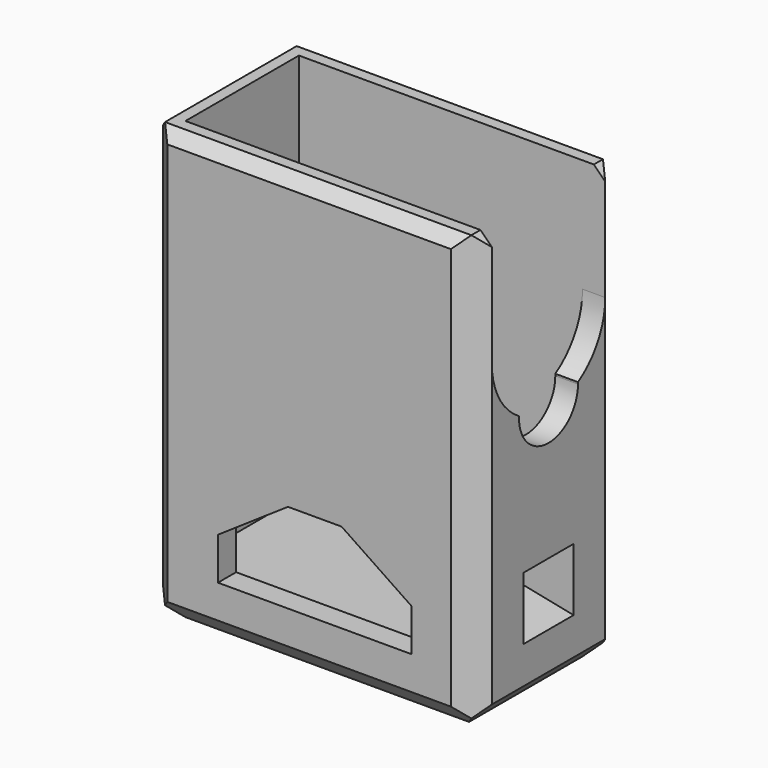
from build123d import *

# Parameters (mm, degrees)
F0_W      = 29
F0_H      = 16.5
F1_DEPTH  = 38.5
F2_T      = -2
F3_DEPTH  = 2.25
F4_SIZE   = 2
F5_SIZE   = 2
F6_SIZE   = 0.99999
F8_DEPTH  = 16.501
F10_DEPTH = 2
F11_R     = 2
F12_DEPTH = 2.001
F13_W     = 7.54
F13_H     = 7.25
F13_R     = 1.1
F14_DEPTH = 6.35
F17_W     = 5.481
F17_H     = 4.583
F15_W     = 5.538
F15_H     = 5.533


# Not quite as in the source:
# - a fillet or chamfer is up to 0.001 mm smaller than in the source, because OpenCascade refuses the exact size


with BuildPart() as f1:
    # F0 (on Top) → F1 (new body)
    with BuildSketch(Plane.XY):
        with Locations((14.5, 8.25)):
            Rectangle(F0_W, F0_H)
    extrude(amount=F1_DEPTH)

    # F2
    f2_openings = [f1.faces().sort_by_distance(p)[0] for p in [
        (14.5, 8.25, 38.5),
    ]]
    offset(amount=F2_T, openings=f2_openings)

    # F3 (add): a face of the model
    f3_faces = [f1.faces().sort_by_distance(p)[0] for p in [
        (14.5, 8.25, 2),
    ]]
    extrude(f3_faces, amount=F3_DEPTH)

    # F4
    f4_edges = [f1.edges().sort_by_distance(p)[0] for p in [
        (29, 0, 19.25),
        (29, 16.5, 19.25),
        (0, 16.5, 19.25),
        (0, 0, 19.25),
    ]]
    chamfer(f4_edges, length=F4_SIZE)

    # F5 (call 1 of 4: OpenCascade refuses the feature's edges together)
    f5_edges = [f1.edges().sort_by_distance(p)[0] for p in [
        (14.5, 16.5, 0),
    ]]
    chamfer(f5_edges, length=F5_SIZE)

    # F5#2 (call 2 of 4)
    f5_2_edges = [f1.edges().sort_by_distance(p)[0] for p in [
        (0, 8.25, 0),
    ]]
    chamfer(f5_2_edges, length=F5_SIZE)

    # F5#3 (call 3 of 4)
    f5_3_edges = [f1.edges().sort_by_distance(p)[0] for p in [
        (14.5, 0, 0),
    ]]
    chamfer(f5_3_edges, length=F5_SIZE)

    # F5#4 (call 4 of 4)
    f5_4_edges = [f1.edges().sort_by_distance(p)[0] for p in [
        (29, 8.25, 0),
    ]]
    chamfer(f5_4_edges, length=F5_SIZE)

    # F6 (size 1 in the source; OpenCascade refuses exactly that, so slightly less here)
    f6_edges = [f1.edges().sort_by_distance(p)[0] for p in [
        (14.5, 16.5, 38.5),
        (0, 8.25, 38.5),
        (14.5, 0, 38.5),
        (29, 8.25, 38.5),
    ]]
    chamfer(f6_edges, length=F6_SIZE)

    # F7 (on face) → F8 (cut, through all)
    with BuildSketch(Plane.XZ):
        Polygon((6.464, 8.664), (6.464, 4.94), (23.536, 4.94), (23.536, 8.664), (17.364, 12.834), (12.635, 12.834), align=None)
    extrude(amount=-F8_DEPTH, mode=Mode.SUBTRACT)

    # F9 (on face) → F10 (cut, through all)
    with BuildSketch(Plane.YZ.offset(29)):
        with BuildLine():
            Line((14.5, 38.5), (2, 38.5))
            Line((2, 38.5), (2, 28.5))
            ThreePointArc((2, 28.5), (8.25, 34.75), (14.5, 28.5))
            Line((14.5, 28.5), (14.5, 38.5))
        make_face()
        with BuildLine():
            ThreePointArc((14.5, 28.5), (8.25, 34.75), (2, 28.5))
            Line((2, 28.5), (14.5, 28.5))
        make_face()
        with BuildLine():
            Line((14.5, 28.5), (2, 28.5))
            ThreePointArc((2, 28.5), (2.8024937382, 25.4361502113), (5.0038961688, 23.1590909091))
            ThreePointArc((5.0038961688, 23.1590909091), (8.25, 26.25), (11.4961038312, 23.1590909091))
            ThreePointArc((11.4961038312, 23.1590909091), (13.6975062618, 25.4361502113), (14.5, 28.5))
        make_face()
        with BuildLine():
            ThreePointArc((11.4961038312, 23.1590909091), (8.25, 26.25), (5.0038961688, 23.1590909091))
            ThreePointArc((5.0038961688, 23.1590909091), (8.25, 22.25), (11.4961038312, 23.1590909091))
        make_face()
        with BuildLine():
            ThreePointArc((11.4961038312, 23.1590909091), (8.25, 22.25), (5.0038961688, 23.1590909091))
            ThreePointArc((5.0038961688, 23.1590909091), (8.1704306945, 19.7509741882), (11.5, 23))
            ThreePointArc((11.5, 23), (11.4990258118, 23.0795693055), (11.4961038312, 23.1590909091))
        make_face()
    extrude(amount=-F10_DEPTH, mode=Mode.SUBTRACT)

    # F11 (on face) → F12 (cut, through all)
    with BuildSketch(Plane.YZ.offset(2)):
        with Locations((8.25, 23)):
            Circle(F11_R)
    extrude(amount=-F12_DEPTH, mode=Mode.SUBTRACT)

    # F13 (on face) → F14 (join)
    with BuildSketch(Plane.YZ.offset(29)):
        with Locations((8.25, 7.875)):
            Rectangle(F13_W, F13_H)
        with Locations((8.25, 9)):
            Circle(F13_R, mode=Mode.SUBTRACT)
    extrude(amount=-F14_DEPTH)

    # F17 (on offset) → F18 section 0
    with BuildSketch(Plane.YZ.offset(24.55)):
        with Locations((8.2215, 8.5135)):
            Rectangle(F17_W, F17_H)
    # F15 (on face) → F18 section 1
    with BuildSketch(Plane.YZ.offset(29)):
        with Locations((8.25, 8.0385)):
            Rectangle(F15_W, F15_H)
    loft(mode=Mode.SUBTRACT)


solid = f1.part
